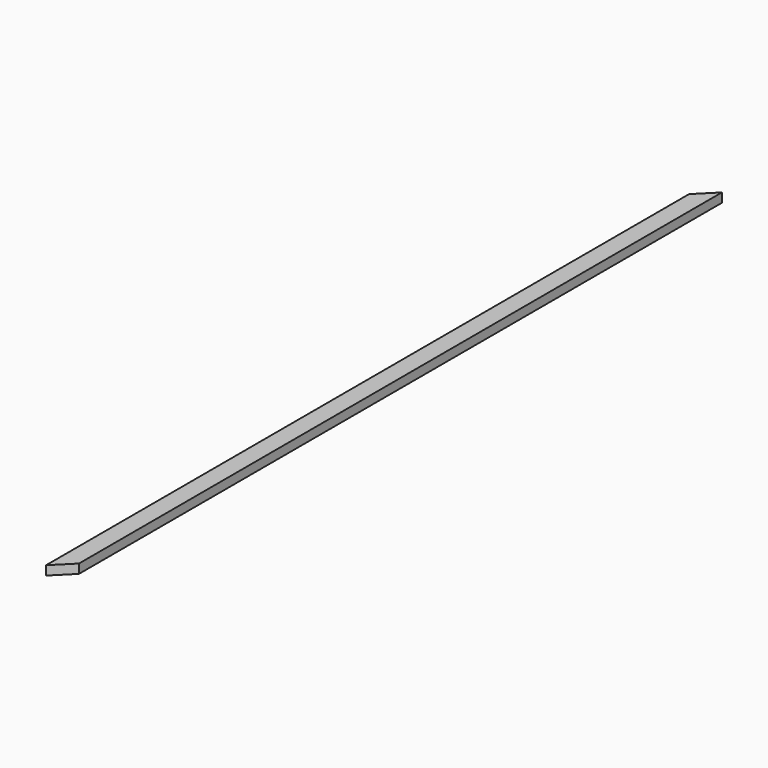
from build123d import *

# Parameters (mm, degrees)
F0_W     = 50.8
F0_H     = 25.4
F1_DEPTH = 2286
F2_SIZE  = 50.79999
F3_SIZE  = 50.79999


# Not quite as in the source:
# - a fillet or chamfer is up to 0.001 mm smaller than in the source, because OpenCascade refuses the exact size


with BuildPart() as f1:
    # F0 (on Front) → F1 (new body)
    with BuildSketch(Plane.XZ):
        with Locations((-48.4498171136, 34.2527418578)):
            Rectangle(F0_W, F0_H)
    extrude(amount=F1_DEPTH)

    # F2 (size 50.8 in the source; OpenCascade refuses exactly that, so slightly less here)
    f2_edges = [f1.edges().sort_by_distance(p)[0] for p in [
        (-23.049817, -2286, 34.252742),
    ]]
    chamfer(f2_edges, length=F2_SIZE)

    # F3 (size 50.8 in the source; OpenCascade refuses exactly that, so slightly less here)
    f3_edges = [f1.edges().sort_by_distance(p)[0] for p in [
        (-73.849817, 0, 34.252742),
    ]]
    chamfer(f3_edges, length=F3_SIZE)


solid = f1.part
